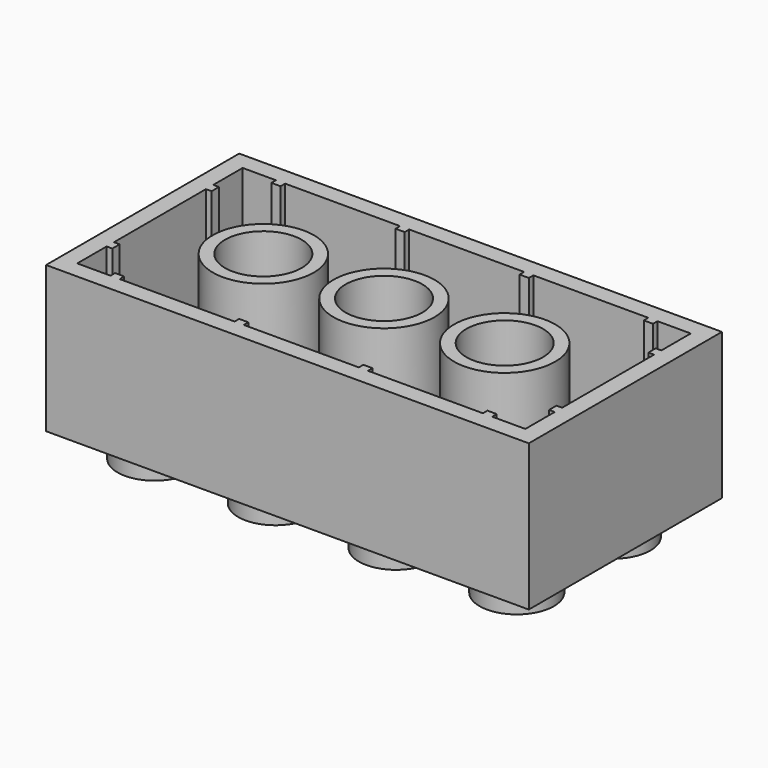
from build123d import *

# Parameters (mm, degrees)
F0_W     = 31.5
F0_H     = 15.75
F0_W_2   = 0.37
F0_H_2   = 0.6
F0_W_3   = 0.6
F0_H_3   = 0.37
F1_DEPTH = 9.55
F0_R     = 3.3
F0_R_2   = 2.5
F2_DEPTH = 1.55
F3_R     = 2.425
F4_DEPTH = 1.9


# Not quite as in the source:
# - a feature names something its author has since deleted; it is built from what else it names


with BuildPart() as f1:
    # F0 (on Top) → F1 (new body)
    with BuildSketch(Plane.XY):
        with Locations((-15.75, 7.875)):
            Rectangle(F0_W, F0_H)
        Polygon((-30.37, 12.225), (-30.37, 14.62), (-28.2, 14.62), (-27.6, 14.62), (-20.1, 14.62), (-19.5, 14.62), (-12, 14.62), (-11.4, 14.62), (-3.9, 14.62), (-3.3, 14.62), (-1.13, 14.62), (-1.13, 12.225), (-1.13, 11.625), (-1.13, 4.125), (-1.13, 3.525), (-1.13, 1.13), (-3.3, 1.13), (-3.9, 1.13), (-11.4, 1.13), (-12, 1.13), (-19.5, 1.13), (-20.1, 1.13), (-27.6, 1.13), (-28.2, 1.13), (-30.37, 1.13), (-30.37, 3.525), (-30.37, 4.125), (-30.37, 11.625), align=None, mode=Mode.SUBTRACT)
        with Locations((-30.185, 11.925)):
            Rectangle(F0_W_2, F0_H_2)
        with Locations((-27.9, 14.435)):
            Rectangle(F0_W_3, F0_H_3)
        with Locations((-19.8, 14.435)):
            Rectangle(F0_W_3, F0_H_3)
        with Locations((-11.7, 14.435)):
            Rectangle(F0_W_3, F0_H_3)
        with Locations((-3.6, 14.435)):
            Rectangle(F0_W_3, F0_H_3)
        with Locations((-1.315, 11.925)):
            Rectangle(F0_W_2, F0_H_2)
        with Locations((-1.315, 3.825)):
            Rectangle(F0_W_2, F0_H_2)
        with Locations((-3.6, 1.315)):
            Rectangle(F0_W_3, F0_H_3)
        with Locations((-11.7, 1.315)):
            Rectangle(F0_W_3, F0_H_3)
        with Locations((-19.8, 1.315)):
            Rectangle(F0_W_3, F0_H_3)
        with Locations((-27.9, 1.315)):
            Rectangle(F0_W_3, F0_H_3)
        with Locations((-30.185, 3.825)):
            Rectangle(F0_W_2, F0_H_2)
    extrude(amount=F1_DEPTH)



with BuildPart() as f1b:
    # F0 (on Top) → F1, piece 2 (new body)
    with BuildSketch(Plane.XY):
        with Locations((-23.625, 7.875)):
            Circle(F0_R)
        with Locations((-23.625, 7.875)):
            Circle(F0_R_2, mode=Mode.SUBTRACT)
    extrude(amount=F1_DEPTH)


with BuildPart() as f1c:
    # F0 (on Top) → F1, piece 3 (new body)
    with BuildSketch(Plane.XY):
        with Locations((-7.875, 7.875)):
            Circle(F0_R)
        with Locations((-7.875, 7.875)):
            Circle(F0_R_2, mode=Mode.SUBTRACT)
    extrude(amount=F1_DEPTH)


with BuildPart() as f1d:
    # F0 (on Top) → F1, piece 4 (new body)
    with BuildSketch(Plane.XY):
        with Locations((-15.75, 7.875)):
            Circle(F0_R)
        with Locations((-15.75, 7.875)):
            Circle(F0_R_2, mode=Mode.SUBTRACT)
    extrude(amount=F1_DEPTH)


with BuildPart() as f1_1:
    add(f1.part)

    add(f1b.part)  # F2 merges F1b

    add(f1c.part)  # F2 merges F1c

    add(f1d.part)  # F2 merges F1d
    # F0 (on Top) → F2 (join)
    with BuildSketch(Plane.XY):
        Polygon((-28.2, 14.62), (-30.37, 14.62), (-30.37, 12.225), (-30, 12.225), (-30, 11.625), (-30.37, 11.625), (-30.37, 4.125), (-30, 4.125), (-30, 3.525), (-30.37, 3.525), (-30.37, 1.13), (-28.2, 1.13), (-28.2, 1.5), (-27.6, 1.5), (-27.6, 1.13), (-20.1, 1.13), (-20.1, 1.5), (-19.5, 1.5), (-19.5, 1.13), (-12, 1.13), (-12, 1.5), (-11.4, 1.5), (-11.4, 1.13), (-3.9, 1.13), (-3.9, 1.5), (-3.3, 1.5), (-3.3, 1.13), (-1.13, 1.13), (-1.13, 3.525), (-1.5, 3.525), (-1.5, 4.125), (-1.13, 4.125), (-1.13, 11.625), (-1.5, 11.625), (-1.5, 12.225), (-1.13, 12.225), (-1.13, 14.62), (-3.3, 14.62), (-3.3, 14.25), (-3.9, 14.25), (-3.9, 14.62), (-11.4, 14.62), (-11.4, 14.25), (-12, 14.25), (-12, 14.62), (-19.5, 14.62), (-19.5, 14.25), (-20.1, 14.25), (-20.1, 14.62), (-27.6, 14.62), (-27.6, 14.25), (-28.2, 14.25), align=None)
        with Locations((-23.625, 7.875)):
            Circle(F0_R, mode=Mode.SUBTRACT)
        with Locations((-15.75, 7.875)):
            Circle(F0_R, mode=Mode.SUBTRACT)
        with Locations((-7.875, 7.875)):
            Circle(F0_R, mode=Mode.SUBTRACT)
        with Locations((-23.625, 7.875)):
            Circle(F0_R_2)
        with Locations((-7.875, 7.875)):
            Circle(F0_R_2)
        with Locations((-15.75, 7.875)):
            Circle(F0_R_2)
    extrude(amount=F2_DEPTH)

    # F3 (on face) → F4 (join)
    with BuildSketch(Plane.XY):
        with Locations((-27.5625, 3.9375)):
            Circle(F3_R)
        with Locations((-11.8125, 3.9375)):
            Circle(F3_R)
        with Locations((-3.9375, 3.9375)):
            Circle(F3_R)
        with Locations((-3.9375, 11.8125)):
            Circle(F3_R)
        with Locations((-11.8125, 11.8125)):
            Circle(F3_R)
        with Locations((-19.6875, 11.8125)):
            Circle(F3_R)
        with Locations((-27.5625, 11.8125)):
            Circle(F3_R)
        with Locations((-19.6875, 3.9375)):
            Circle(F3_R)
    extrude(amount=-F4_DEPTH)


solid = f1_1.part
